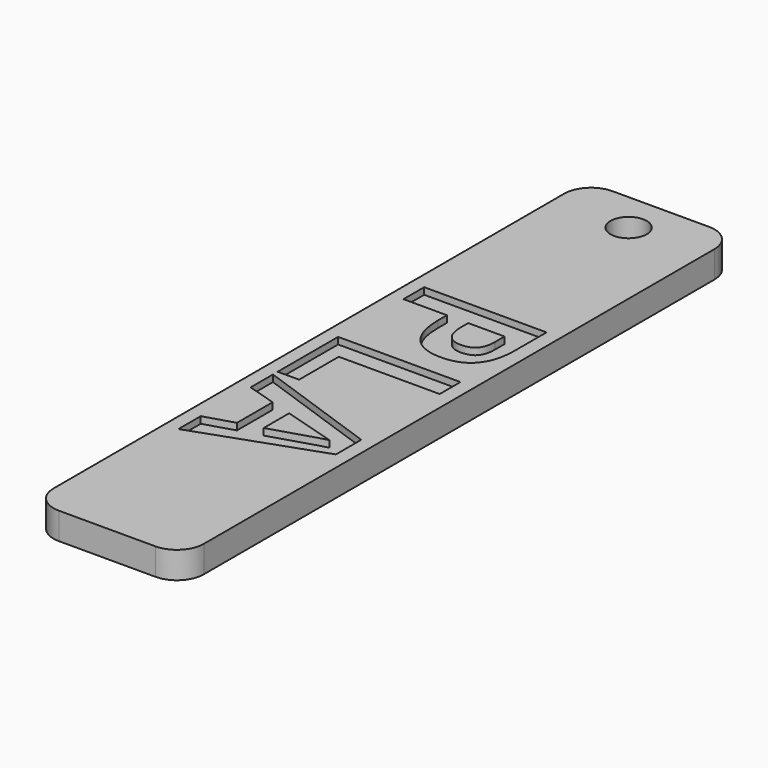
from build123d import *

# Parameters (mm, degrees)
F0_W         = 11.2
F0_H         = 51.6
F0_R         = 1.35
F0_TEXT_SIZE = 12.7777777778
F1_DEPTH     = 2
F2_DEPTH     = 0.5
F3_R         = 2


# Not quite as in the source:
# - a feature names something its author has since deleted; it is built from what else it names
# - Text() gives the source's letters only with a copy of the font that has no kerning and outlines rounded to 1/6400 em; it was checked with that copy


with BuildPart() as f1:
    # F0 (on Top) → F1 (new body)
    with BuildSketch(Plane.XY):
        with Locations((-43.6647401989, 54.4962232466)):
            Rectangle(F0_W, F0_H)
        Polygon((-48.2647401989, 41.0804246355), (-48.2647401989, 43.1647996355), (-46.0925179766, 43.82565033), (-46.0925179766, 47.1518656077), (-48.2647401989, 47.8127163022), (-48.2647401989, 49.8970913022), (-39.1046707544, 46.6766919966), (-39.1046707544, 44.3128031077), align=None, mode=Mode.SUBTRACT)
        Polygon((-48.2647401989, 50.3343308855), (-48.2647401989, 55.9685322744), (-39.1426047822, 55.9685322744), (-39.1426047822, 54.0338968577), (-46.6675179766, 54.0338968577), (-46.6675179766, 50.3343308855), align=None, mode=Mode.SUBTRACT)
        with BuildLine():
            add(Edge.make_bspline(
                [(-39.8573617266, 58.5550340105), (-40.5721186711, 57.6915357466), (-41.9876568655, 57.6915357466)],
                knots=[0, 0, 0, 1, 1, 1], degree=2))
            add(Edge.make_bspline(
                [(-41.9876568655, 57.6915357466), (-43.4610943655, 57.6915357466), (-44.2407384627, 58.6119350522)],
                knots=[0, 0, 0, 1, 1, 1], degree=2))
            add(Edge.make_bspline(
                [(-44.2407384627, 58.6119350522), (-45.02038256, 59.5323343577), (-45.02038256, 61.2293829688)],
                knots=[0, 0, 0, 1, 1, 1], degree=2))
            Line((-45.02038256, 61.2293829688), (-45.02038256, 62.0579419966))
            Line((-45.02038256, 62.0579419966), (-48.2647401989, 62.0579419966))
            Line((-48.2647401989, 62.0579419966), (-48.2647401989, 63.9925774133))
            Line((-48.2647401989, 63.9925774133), (-39.1426047822, 63.9925774133))
            Line((-39.1426047822, 63.9925774133), (-39.1426047822, 61.0796433855))
            add(Edge.make_bspline(
                [(-39.1426047822, 61.0796433855), (-39.1426047822, 59.4185322744), (-39.8573617266, 58.5550340105)],
                knots=[0, 0, 0, 1, 1, 1], degree=2))
        make_face(mode=Mode.SUBTRACT)
        with Locations((-43.6647401989, 77.2962232466)):
            Circle(F0_R, mode=Mode.SUBTRACT)
        with Locations(Location((-48.2647401989, 65.1405808855), (0, 0, -90))):
            Text('PLA', F0_TEXT_SIZE, font='Open Sans', font_style=FontStyle.BOLD, text_align=(TextAlign.LEFT, TextAlign.BOTTOM))
        with BuildLine():
            Line((-40.7278478377, 62.0579419966), (-43.4351395044, 62.0579419966))
            Line((-43.4351395044, 62.0579419966), (-43.4351395044, 61.4210496355))
            add(Edge.make_bspline(
                [(-43.4351395044, 61.4210496355), (-43.4351395044, 60.5305982466), (-43.0827523516, 60.08736908)],
                knots=[0, 0, 0, 1, 1, 1], degree=2))
            add(Edge.make_bspline(
                [(-43.0827523516, 60.08736908), (-42.7303651989, 59.6441399133), (-42.0575353377, 59.6441399133)],
                knots=[0, 0, 0, 1, 1, 1], degree=2))
            add(Edge.make_bspline(
                [(-42.0575353377, 59.6441399133), (-41.3767193655, 59.6441399133), (-41.0522836016, 60.01549408)],
                knots=[0, 0, 0, 1, 1, 1], degree=2))
            add(Edge.make_bspline(
                [(-41.0522836016, 60.01549408), (-40.7278478377, 60.3868482466), (-40.7278478377, 61.1794697744)],
                knots=[0, 0, 0, 1, 1, 1], degree=2))
            Line((-40.7278478377, 61.1794697744), (-40.7278478377, 62.0579419966))
        make_face()
        with BuildLine():
            Line((-44.4713374211, 46.66471283), (-44.4713374211, 44.2888447744))
            add(Edge.make_bspline(
                [(-44.4713374211, 44.2888447744), (-41.5204693655, 45.2052510244), (-41.1331429766, 45.3210496355)],
                knots=[0, 0, 0, 1, 1, 1], degree=2))
            add(Edge.make_bspline(
                [(-41.1331429766, 45.3210496355), (-40.7458165877, 45.4368482466), (-40.5222054766, 45.4867614411)],
                knots=[0, 0, 0, 1, 1, 1], degree=2))
            add(Edge.make_bspline(
                [(-40.5222054766, 45.4867614411), (-41.3208165877, 45.6924038022), (-44.4713374211, 46.66471283)],
                knots=[0, 0, 0, 1, 1, 1], degree=2))
        make_face()
    extrude(amount=-F1_DEPTH)

    # F0 (on Top) → F2 (cut)
    with BuildSketch(Plane.XY):
        with Locations(Location((-48.2647401989, 65.1405808855), (0, 0, -90))):
            Text('PLA', F0_TEXT_SIZE, font='Open Sans', font_style=FontStyle.BOLD, text_align=(TextAlign.LEFT, TextAlign.BOTTOM))
    extrude(amount=-F2_DEPTH, mode=Mode.SUBTRACT)

    # F3
    f3_edges = [f1.edges().sort_by_distance(p)[0] for p in [
        (-49.26474, 80.296223, -1),
        (-38.06474, 80.296223, -1),
        (-38.06474, 28.696223, -1),
        (-49.26474, 28.696223, -1),
    ]]
    fillet(f3_edges, radius=F3_R)


solid = f1.part
